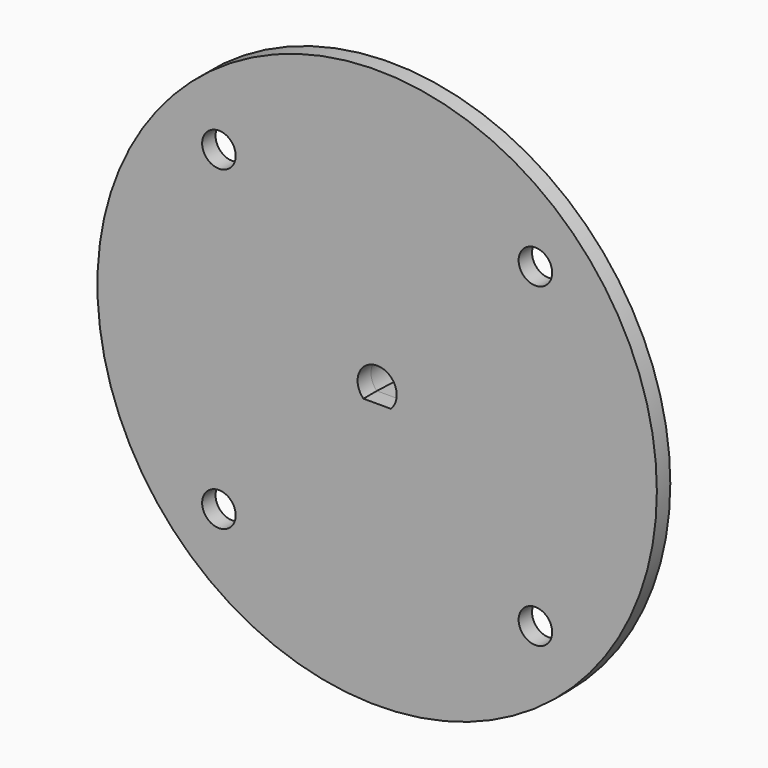
from build123d import *

# Parameters (mm, degrees)
F0_R                   = 7.25
F1_DEPTH               = 10
DRAFT_F1_DRAFTED_ANGLE = 3
F0_R_2                 = 25
F0_R_3                 = 1.5
F2_DEPTH               = 1.5


# Not quite as in the source:
# - an extrude with a draft is written as a straight extrude whose walls are then drafted


with BuildPart() as f1:
    # F0 (on Front) → F1 (new body)
    with BuildSketch(Plane.XZ):
        Circle(F0_R)
        with BuildLine():
            Line((1.2247448714, -1.25), (-1.2247448714, -1.25))
            ThreePointArc((-1.2247448714, -1.25), (0, 1.75), (1.2247448714, -1.25))
        make_face(mode=Mode.SUBTRACT)
    extrude(amount=-F1_DEPTH)

    # draft_F1_drafted
    draft_f1_drafted_walls = [f1.faces().sort_by_distance(p)[0] for p in [
        (-7.25, 6.6666666667, 0),
        (0, 6.6666666667, -1.25),
        (0, 6.6666666667, 1.75),
    ]]
    draft(draft_f1_drafted_walls, neutral_plane=Plane(origin=(0, 0, 0), x_dir=(1, 0, 0), z_dir=(0, 1, 0)), angle=DRAFT_F1_DRAFTED_ANGLE)

    # F0 (on Front) → F2 (join)
    with BuildSketch(Plane.XZ):
        Circle(F0_R_2)
        with Locations((-14.1421356237, -14.1421356237)):
            Circle(F0_R_3, mode=Mode.SUBTRACT)
        with Locations((14.1421356237, -14.1421356237)):
            Circle(F0_R_3, mode=Mode.SUBTRACT)
        with Locations((-14.1421356237, 14.1421356237)):
            Circle(F0_R_3, mode=Mode.SUBTRACT)
        Circle(F0_R, mode=Mode.SUBTRACT)
        with Locations((14.1421356237, 14.1421356237)):
            Circle(F0_R_3, mode=Mode.SUBTRACT)
        Circle(F0_R)
        with BuildLine():
            Line((1.2247448714, -1.25), (-1.2247448714, -1.25))
            ThreePointArc((-1.2247448714, -1.25), (0, 1.75), (1.2247448714, -1.25))
        make_face(mode=Mode.SUBTRACT)
    extrude(amount=F2_DEPTH)


solid = f1.part
